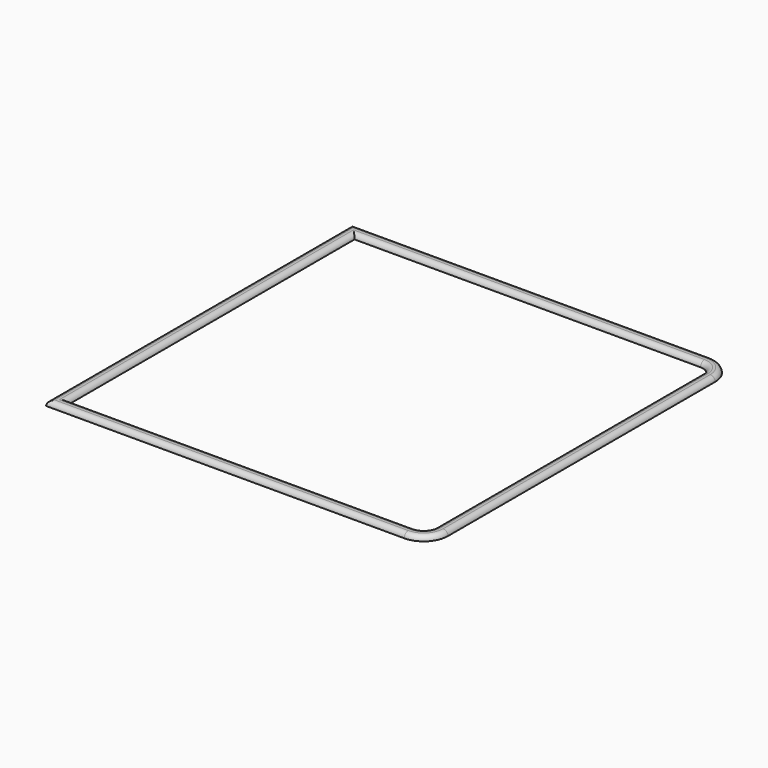
from build123d import *

# Parameters (mm, degrees)
F0_W     = 200
F0_H     = 200
F1_DEPTH = 2.54
F2_R     = 12.7
F4_DEPTH = 2.541
F5_R     = 2.53999


# Not quite as in the source:
# - a fillet or chamfer is up to 0.001 mm smaller than in the source, because OpenCascade refuses the exact size


with BuildPart() as f1:
    # F0 (on Top) → F1 (new body)
    with BuildSketch(Plane.XY):
        with Locations((100, 100)):
            Rectangle(F0_W, F0_H)
    extrude(amount=F1_DEPTH)

    # F2
    f2_edges = [f1.edges().sort_by_distance(p)[0] for p in [
        (200, 0, 1.27),
        (200, 200, 1.27),
    ]]
    fillet(f2_edges, radius=F2_R)

    # F3 (on face) → F4 (cut, through all)
    with BuildSketch(Plane.XY.offset(2.54)):
        with BuildLine():
            Line((6.35, 193.65), (6.35, 6.35))
            Line((6.35, 6.35), (187.3, 6.35))
            ThreePointArc((187.3, 6.35), (191.7901280605, 8.2098719395), (193.65, 12.7))
            Line((193.65, 12.7), (193.65, 187.3))
            ThreePointArc((193.65, 187.3), (191.7901280605, 191.7901280605), (187.3, 193.65))
            Line((187.3, 193.65), (6.35, 193.65))
        make_face()
    extrude(amount=-F4_DEPTH, mode=Mode.SUBTRACT)

    # F5 (radius 2.54 in the source; OpenCascade refuses exactly that, so slightly less here)
    f5_edges = [f1.edges().sort_by_distance(p)[0] for p in [
        (96.825, 193.65, 2.54),
        (6.35, 100, 2.54),
        (196.280256, 196.280256, 2.54),
        (0, 100, 2.54),
    ]]
    fillet(f5_edges, radius=F5_R)


solid = f1.part
